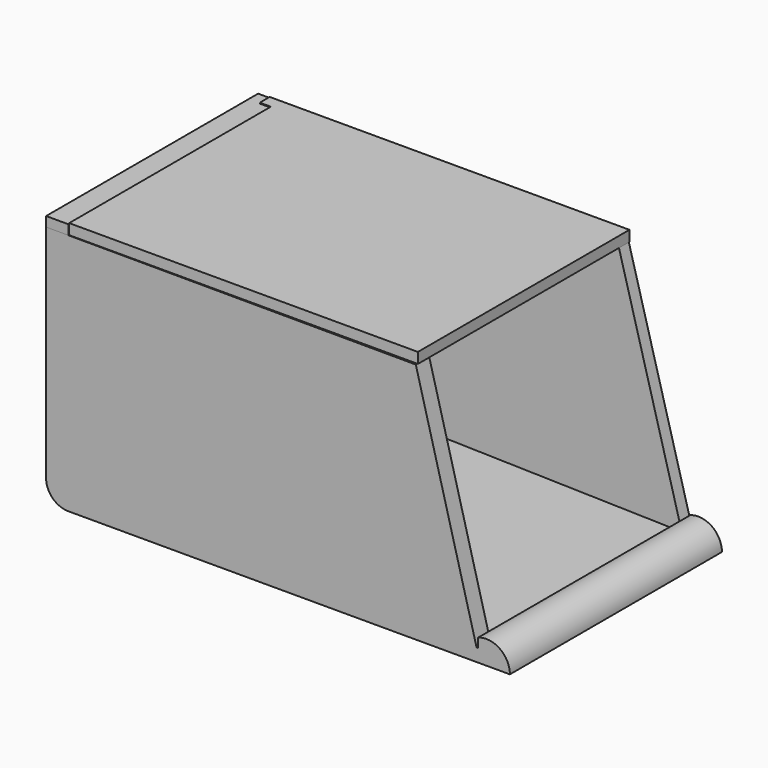
from build123d import *

# Parameters (mm, degrees)
F1_DEPTH      = 76.2
F3_DEPTH      = 3.556
F5_DEPTH      = 5.334
F6_DEPTH      = 4.826
F8_DEPTH      = 3.048
F9_DEPTH      = 2.794
F10_TEXT_SIZE = 8.3122855156
F11_DEPTH     = 2.032


# Not quite as in the source:
# - Text() gives the source's letters only with a copy of the font that has no kerning and outlines rounded to 1/6400 em; it was checked with that copy


with BuildPart() as f1:
    # F0 (on Front) → F1 (new body)
    with BuildSketch(Plane.XZ):
        with BuildLine():
            Line((-13.954042569, 51.9836902678), (-20.4556323588, 51.9836902678))
            Line((-20.4556323588, 51.9836902678), (-20.4556323588, -11.5163097322))
            ThreePointArc((-20.4556323588, -11.5163097322), (-18.5957604193, -16.0064377927), (-14.1056323588, -17.8663097322))
            Line((-14.1056323588, -17.8663097322), (112.8943676412, -17.8663097322))
            ThreePointArc((112.8943676412, -17.8663097322), (109.9933987064, -12.3107724247), (103.7766113877, -11.5163097322))
            Line((103.7766113877, -11.5163097322), (103.7766113877, -14.1639700159))
            Line((103.7766113877, -14.1639700159), (-7.7404552858, -11.5163097322))
            ThreePointArc((-7.7404552858, -11.5163097322), (-12.2359396447, -9.6510750972), (-14.0904371918, -5.1511507964))
            Line((-14.0904371918, -5.1511507964), (-13.954042569, 51.9836902678))
        make_face()
    extrude(amount=F1_DEPTH)

    # F2 (on Front) → F3 (join)
    with BuildSketch(Plane.XZ):
        Polygon((86.0033035278, 52.3340329528), (-17.1271105215, 52.3340329528), (-17.0558914542, -13.0849499255), (104.3305322528, -14.6893328056), align=None)
    extrude(amount=F3_DEPTH)

    # F4 (on face) → F5 (join)
    with BuildSketch(Plane.XZ.offset(76.2)):
        with BuildLine():
            Line((-14.0904371918, -5.1511507964), (-13.954042569, 51.9836902678))
            Line((-13.954042569, 51.9836902678), (-15.8363445937, 48.6750783097))
            Line((-15.8363445937, 48.6750783097), (-16.7530961335, -14.1639700159))
            Line((-16.7530961335, -14.1639700159), (103.7766113877, -15.9223638475))
            Line((103.7766113877, -15.9223638475), (103.3075028276, -14.1528323476))
            Line((103.3075028276, -14.1528323476), (-7.7404552858, -11.5163097322))
            ThreePointArc((-7.7404552858, -11.5163097322), (-12.2359396447, -9.6510750972), (-14.0904371918, -5.1511507964))
        make_face()
    extrude(amount=-F5_DEPTH)

    # F4 (on face) → F6 (join)
    with BuildSketch(Plane.XZ.offset(76.2)):
        Polygon((85.8376501192, 51.7454634691), (-13.954042569, 51.9836902678), (-15.8363445937, 48.6750783097), (-16.7530961335, -14.1639700159), (103.7766113877, -15.9223638475), align=None)
    extrude(amount=-F6_DEPTH)


with BuildPart() as f8:
    # F7 (on face) → F8 (new body)
    with BuildSketch(Plane.XY.offset(51.9836902678)):
        Polygon((86.3065868616, 0), (-17.1267291172, 0), (-17.1267291172, -3.556), (-13.954042569, -3.556), (-13.954042569, -71.374), (-13.954042569, -76.0283172131), (86.3065868616, -76.0283172131), align=None)
    extrude(amount=F8_DEPTH)


with BuildPart() as f9:
    # F9 (new): a face of the model
    f9_faces = [f1.part.faces().sort_by_distance(p)[0] for p in [
        (-17.2436248011, -38.946425119, 51.9836902678),
    ]]
    extrude(f9_faces, amount=F9_DEPTH)


with BuildPart() as f1_1:
    add(f1.part)

    # F10 (on face) → F11 (join)
    with BuildSketch(Plane(origin=(0, 0, 0), x_dir=(-1, 0, 0), z_dir=(0, 1, 0))):
        with Locations((-59.9257238209, 13.7624321505)):
            Text('Blue Team pd 3', F10_TEXT_SIZE, font='Open Sans', text_align=(TextAlign.LEFT, TextAlign.BOTTOM))
    extrude(amount=F11_DEPTH)


solid = Compound([f8.part, f9.part, f1_1.part])
